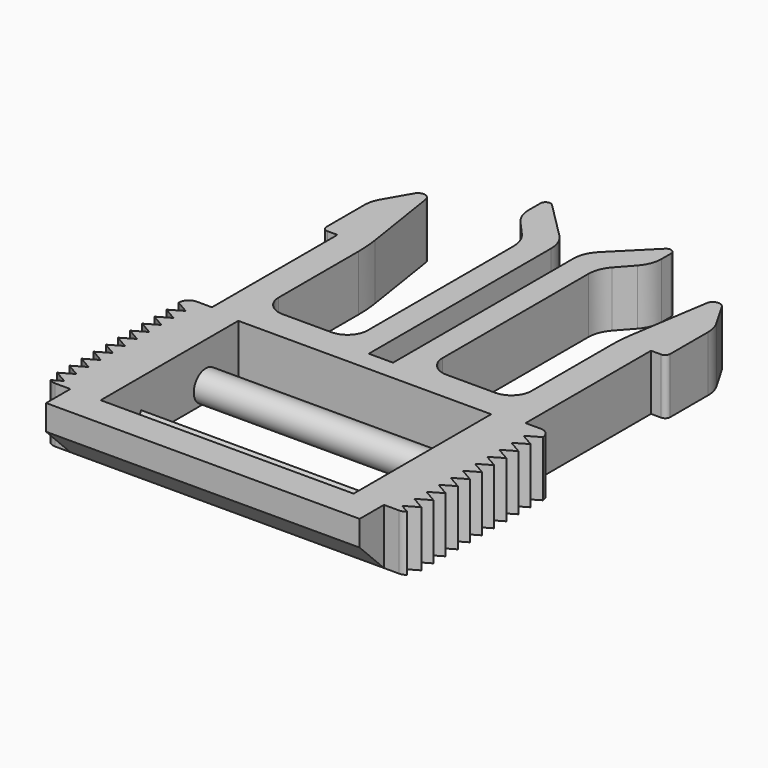
from build123d import *

# Parameters (mm, degrees)
F0_W      = 25
F0_H      = 17
F1_DEPTH  = 5.5
F3_DEPTH  = 25
F5_DEPTH  = 32.501
F7_DEPTH  = 5.5
F9_DEPTH  = 5.501
F12_SCALE = 0.5


with BuildPart() as f1:
    # F0 (on Top) → F1 (new body)
    with BuildSketch(Plane.XY):
        with BuildLine():
            Line((-15.5, -24.3527164447), (15.5, -24.3527164447))
            Line((15.5, -24.3527164447), (15.5, 11.6472835553))
            Line((15.5, 11.6472835553), (16.5, 11.6472835553))
            ThreePointArc((16.5, 11.6472835553), (16.8535533906, 11.7937301647), (17, 12.1472835553))
            Line((17, 12.1472835553), (17, 16.843435978))
            ThreePointArc((17, 16.843435978), (16.8977774789, 17.6198931134), (16.5980762114, 18.343435978))
            Line((16.5980762114, 18.343435978), (15.1841674029, 20.7923978715))
            ThreePointArc((15.1841674029, 20.7923978715), (14.4494876631, 21.1305094363), (13.8862846459, 20.5500991403))
            Line((13.8862846459, 20.5500991403), (12.678607693, 12.7943144757))
            ThreePointArc((12.678607693, 12.7943144757), (12.5447185816, 11.6438227741), (12.5, 10.4864301451))
            Line((12.5, 10.4864301451), (12.5, 0.6472835553))
            ThreePointArc((12.5, 0.6472835553), (11.9142135624, -0.766930007), (10.5, -1.3527164447))
            Line((10.5, -1.3527164447), (5.7, -1.3527164447))
            ThreePointArc((5.7, -1.3527164447), (4.2857864376, -0.766930007), (3.7, 0.6472835553))
            Line((3.7, 0.6472835553), (3.7, 18.6472835553))
            ThreePointArc((3.7, 18.6472835553), (3.8975072906, 19.7178136174), (4.4640230758, 20.6473853514))
            Line((4.4640230758, 20.6473853514), (5.7959697488, 22.1364105755))
            ThreePointArc((5.7959697488, 22.1364105755), (6.362485534, 23.0659823095), (6.5599928246, 24.1365123716))
            Line((6.5599928246, 24.1365123716), (6.5599928246, 25.3001695988))
            ThreePointArc((6.5599928246, 25.3001695988), (6.2513345408, 25.762109365), (5.706439434, 25.6537229894))
            Line((5.706439434, 25.6537229894), (2.0786796564, 22.0259632118))
            ThreePointArc((2.0786796564, 22.0259632118), (1.4283614025, 21.0526931653), (1.2, 19.9046428682))
            Line((1.2, 19.9046428682), (1.2, -2.3527164447))
            Line((1.2, -2.3527164447), (-1.2, -2.3527164447))
            Line((-1.2, -2.3527164447), (-1.2, 20.1675462621))
            ThreePointArc((-1.2, 20.1675462621), (-1.4283614025, 21.3155965592), (-2.0786796564, 22.2888666056))
            Line((-2.0786796564, 22.2888666056), (-5.706439434, 25.9166263832))
            ThreePointArc((-5.706439434, 25.9166263832), (-6.2513345408, 26.0250127589), (-6.5599928246, 25.5630729926))
            Line((-6.5599928246, 25.5630729926), (-6.5599928246, 24.1365123716))
            ThreePointArc((-6.5599928246, 24.1365123716), (-6.362485534, 23.0659823095), (-5.7959697488, 22.1364105755))
            Line((-5.7959697488, 22.1364105755), (-4.4640230758, 20.6473853514))
            ThreePointArc((-4.4640230758, 20.6473853514), (-3.8975072906, 19.7178136174), (-3.7, 18.6472835553))
            Line((-3.7, 18.6472835553), (-3.7, 0.6472835553))
            ThreePointArc((-3.7, 0.6472835553), (-4.2857864376, -0.766930007), (-5.7, -1.3527164447))
            Line((-5.7, -1.3527164447), (-10.5, -1.3527164447))
            ThreePointArc((-10.5, -1.3527164447), (-11.9142135624, -0.766930007), (-12.5, 0.6472835553))
            Line((-12.5, 0.6472835553), (-12.5, 10.4864301451))
            ThreePointArc((-12.5, 10.4864301451), (-12.5447185816, 11.6438227741), (-12.678607693, 12.7943144757))
            Line((-12.678607693, 12.7943144757), (-13.8862846459, 20.5500991403))
            ThreePointArc((-13.8862846459, 20.5500991403), (-14.4494876631, 21.1305094363), (-15.1841674029, 20.7923978715))
            Line((-15.1841674029, 20.7923978715), (-16.5980762114, 18.343435978))
            ThreePointArc((-16.5980762114, 18.343435978), (-16.8977774789, 17.6198931134), (-17, 16.843435978))
            Line((-17, 16.843435978), (-17, 12.1472835553))
            ThreePointArc((-17, 12.1472835553), (-16.8535533906, 11.7937301647), (-16.5, 11.6472835553))
            Line((-16.5, 11.6472835553), (-15.5, 11.6472835553))
            Line((-15.5, 11.6472835553), (-15.5, -24.3527164447))
        make_face()
        with Locations((0, -12.8527164447)):
            Rectangle(F0_W, F0_H, mode=Mode.SUBTRACT)
    extrude(amount=F1_DEPTH)

    # F2 (on face) → F3 (join)
    with BuildSketch(Plane.YZ.offset(-12.5)):
        Polygon((-14.8527164447, 0), (-16.3527164447, 2.5980762114), (-17.8527164447, 0), align=None)
        with BuildLine():
            ThreePointArc((-6.8527164447, 1.5), (-9.4133766164, 2.5606601718), (-8.3527164447, 0))
            ThreePointArc((-8.3527164447, 0), (-7.2920562729, 0.4393398282), (-6.8527164447, 1.5))
        make_face()
    extrude(amount=F3_DEPTH)

    # F4 (on face) → F5 (cut, through all)
    with BuildSketch(Plane.YZ.offset(15.5)):
        Polygon((-24.3527164447, 0), (-21.3527164447, 0), (-24.3527164447, 3), align=None)
    extrude(amount=-F5_DEPTH, mode=Mode.SUBTRACT)



with BuildPart() as f7:
    # F6 (on face) → F7 (new body, through all)
    with BuildSketch(Plane.XY.offset(5.5)):
        with BuildLine():
            Line((17, -3.8527164447), (15.5, -3.8527164447))
            Line((15.5, -3.8527164447), (15.5, -21.3527164447))
            Line((15.5, -21.3527164447), (17, -21.3527164447))
            ThreePointArc((17, -21.3527164447), (17.7071067812, -21.0598232258), (18, -20.3527164447))
            Line((18, -20.3527164447), (18, -4.8527164447))
            ThreePointArc((18, -4.8527164447), (17.7071067812, -4.1456096635), (17, -3.8527164447))
        make_face()
    extrude(amount=-F7_DEPTH)

    # F8 (on face) → F9 (cut, through all)
    with BuildSketch(Plane.XY.offset(5.5)):
        Polygon((18, -6.3527164447), (18, -4.8527164447), (16.7009618943, -5.6027164447), align=None)
        Polygon((18, -21.3527164447), (18, -19.8527164447), (16.7009618943, -20.6027164447), align=None)
        Polygon((18, -19.8527164447), (18, -18.3527164447), (16.7009618943, -19.1027164447), align=None)
        Polygon((18, -18.3527164447), (18, -16.8527164447), (16.7009618943, -17.6027164447), align=None)
        Polygon((18, -16.8527164447), (18, -15.3527164447), (16.7009618943, -16.1027164447), align=None)
        Polygon((18, -15.3527164447), (18, -13.8527164447), (16.7009618943, -14.6027164447), align=None)
        Polygon((18, -13.8527164447), (18, -12.3527164447), (16.7009618943, -13.1027164447), align=None)
        Polygon((18, -12.3527164447), (18, -10.8527164447), (16.7009618943, -11.6027164447), align=None)
        Polygon((18, -10.8527164447), (18, -9.3527164447), (16.7009618943, -10.1027164447), align=None)
        Polygon((18, -9.3527164447), (18, -7.8527164447), (16.7009618943, -8.6027164447), align=None)
        Polygon((18, -7.8527164447), (18, -6.3527164447), (16.7009618943, -7.1027164447), align=None)
    extrude(amount=-F9_DEPTH, mode=Mode.SUBTRACT)


with BuildPart() as f1_1:
    add(f1.part)

    add(f7.part)  # F11 merges F7
    # F11: F7 across plane
    add(f7.part.mirror(Plane(origin=(0, -5.9573676074, 2.7906976744), x_dir=(0, 1, 0), z_dir=(1, 0, 0))))


with BuildPart() as f1_2:
    # F12: moved
    add(f1_1.part.scale(F12_SCALE).moved(Location((0, 13.9478668571, 0))))


solid = f1_2.part
